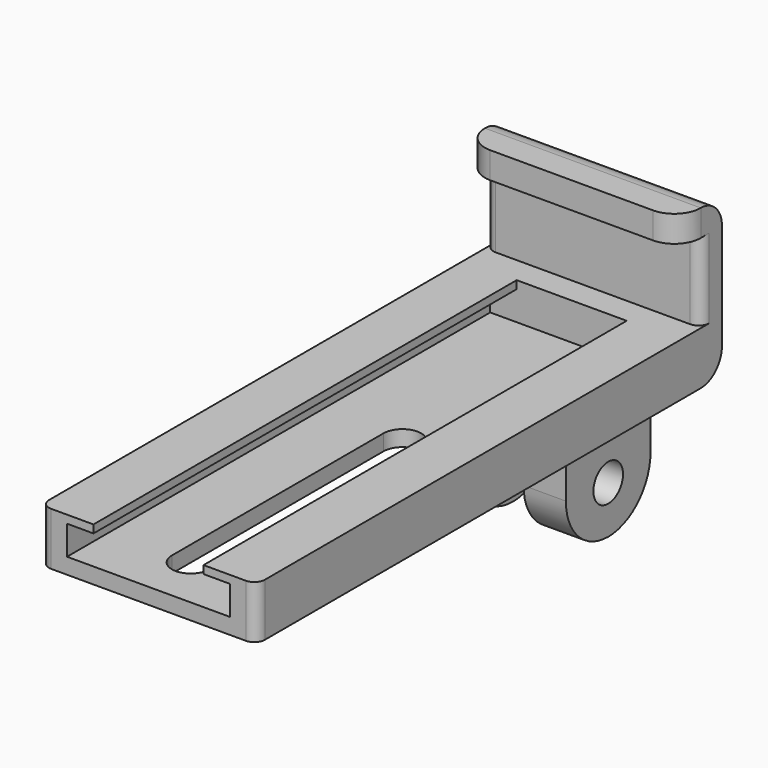
from build123d import *

# Parameters (mm, degrees)
F0_W      = 10
F0_H      = 100
F1_DEPTH  = 10
F0_W_2    = 20.8
F2_DEPTH  = 5
F3_W      = 40.8
F3_H      = 5
F4_DEPTH  = 15
F5_W      = 40.8
F5_H      = 10
F6_DEPTH  = 5
F7_W      = 8
F7_H      = 20
F8_DEPTH  = 22
F9_R      = 3.5
F10_DEPTH = 33.401
F11_DEPTH = 5
F12_R     = 9.99999
F13_R     = 4.99999
F14_R     = 2
F15_W     = 100
F15_H     = 3.5
F16_DEPTH = 5
F17_W     = 100
F17_H     = 3.5
F18_DEPTH = 5
F19_DEPTH = 2


# Not quite as in the source:
# - a fillet or chamfer is up to 0.001 mm smaller than in the source, because OpenCascade refuses the exact size


with BuildPart() as f1:
    # F0 (on Top) → F1 (new body)
    with BuildSketch(Plane.XY):
        with Locations((-15.4, 0)):
            Rectangle(F0_W, F0_H)
        Polygon((-10.4, 50), (10.4, 50), (20.4, 50), (20.4, 60), (-20.4, 60), (-20.4, 50), align=None)
        with Locations((15.4, 0)):
            Rectangle(F0_W, F0_H)
    extrude(amount=F1_DEPTH)

    # F0 (on Top) → F2 (join)
    with BuildSketch(Plane.XY):
        Rectangle(F0_W_2, F0_H)
        with BuildLine():
            Line((3.5661098082, 10), (3.5661098082, -40))
            ThreePointArc((3.5661098082, -40), (0, -43.5661098082), (-3.5661098082, -40))
            Line((-3.5661098082, -40), (-3.5661098082, 10))
            ThreePointArc((-3.5661098082, 10), (0, 13.5661098082), (3.5661098082, 10))
        make_face(mode=Mode.SUBTRACT)
    extrude(amount=F2_DEPTH)

    # F3 (on face) → F4 (join)
    with BuildSketch(Plane.XY.offset(10)):
        with Locations((0, 57.5)):
            Rectangle(F3_W, F3_H)
    extrude(amount=F4_DEPTH)

    # F5 (on face) → F6 (join)
    with BuildSketch(Plane.XY.offset(25)):
        with Locations((0, 55)):
            Rectangle(F5_W, F5_H)
    extrude(amount=F6_DEPTH)

    # F7 (on face) → F8 (join)
    with BuildSketch(Plane(origin=(0, 0, 0), x_dir=(1, 0, 0), z_dir=(0, 0, -1))):
        with Locations((9, -42.3806495965)):
            Rectangle(F7_W, F7_H)
        with Locations((-9, -42.3806495965)):
            Rectangle(F7_W, F7_H)
    extrude(amount=F8_DEPTH)

    # F9 (on face) → F10 (cut, through all)
    with BuildSketch(Plane(origin=(-13, 0, 0), x_dir=(0, -1, 0), z_dir=(-1, 0, 0))):
        with Locations((-42.3806495965, -13)):
            Circle(F9_R)
    extrude(amount=-F10_DEPTH, mode=Mode.SUBTRACT)

    # F9 (on face) → F11 (cut)
    with BuildSketch(Plane(origin=(-13, 0, 0), x_dir=(0, -1, 0), z_dir=(-1, 0, 0))):
        Polygon((-39.0320180352, -7.2), (-45.7292811578, -7.2), (-49.0779127191, -13), (-45.7292811578, -18.8), (-39.0320180352, -18.8), (-35.6833864739, -13), align=None)
        with Locations((-42.3806495965, -13)):
            Circle(F9_R, mode=Mode.SUBTRACT)
    extrude(amount=-F11_DEPTH, mode=Mode.SUBTRACT)

    # F12 (radius 10 in the source; OpenCascade refuses exactly that, so slightly less here)
    f12_edges = [f1.edges().sort_by_distance(p)[0] for p in [
        (-9, 52.38065, -22),
        (9, 52.38065, -22),
        (9, 32.38065, -22),
        (-9, 32.38065, -22),
    ]]
    fillet(f12_edges, radius=F12_R)

    # F13 (radius 5 in the source; OpenCascade refuses exactly that, so slightly less here)
    f13_edges = [f1.edges().sort_by_distance(p)[0] for p in [
        (-20.4, 50, 27.5),
        (20.4, 50, 27.5),
        (0, 60, 30),
        (0, 60, 0),
    ]]
    fillet(f13_edges, radius=F13_R)

    # F14
    f14_edges = [f1.edges().sort_by_distance(p)[0] for p in [
        (-20.4, 55, 17.5),
        (20.4, 55, 17.5),
        (-20.4, -50, 5),
        (20.4, -50, 5),
    ]]
    fillet(f14_edges, radius=F14_R)

    # F15 (on face) → F16 (cut)
    with BuildSketch(Plane.YZ.offset(-10.4)):
        with Locations((0, 6.75)):
            Rectangle(F15_W, F15_H)
    extrude(amount=-F16_DEPTH, mode=Mode.SUBTRACT)

    # F17 (on face) → F18 (cut)
    with BuildSketch(Plane(origin=(10.4, 0, 0), x_dir=(0, -1, 0), z_dir=(-1, 0, 0))):
        with Locations((0, 6.75)):
            Rectangle(F17_W, F17_H)
    extrude(amount=-F18_DEPTH, mode=Mode.SUBTRACT)

    # F19 (cut): a face of the model
    f19_faces = [f1.faces().sort_by_distance(p)[0] for p in [
        (0, 48.9536425085, 5),
    ]]
    extrude(f19_faces, amount=-F19_DEPTH, mode=Mode.SUBTRACT)


solid = f1.part
